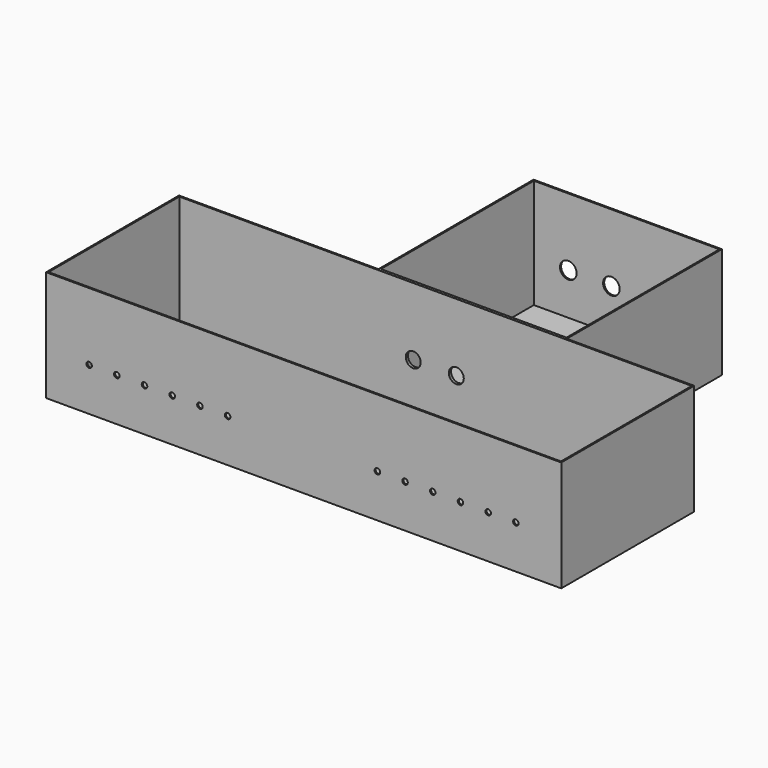
from build123d import *

# Parameters (mm, degrees)
F0_W      = 930
F0_H      = 300
F2_DEPTH  = 200
F3_T      = -2.5
F1_W      = 340
F1_H      = 350
F4_DEPTH  = 200
F5_T      = -2.5
F6_R      = 5
F7_DEPTH  = 25
F8_R      = 13.5
F9_DEPTH  = 25
F10_R     = 15
F11_DEPTH = 25


# Not quite as in the source:
# - a feature names something its author has since deleted; it is built from what else it names


with BuildPart() as f2:
    # F0 (on Top) → F2 (new body)
    with BuildSketch(Plane.XY):
        Rectangle(F0_W, F0_H)
    extrude(amount=F2_DEPTH)

    # F3
    f3_openings = [f2.faces().sort_by_distance(p)[0] for p in [
        (0, 0, 200),
    ]]
    offset(amount=F3_T, openings=f3_openings)

    # F6 (on face) → F7 (cut)
    with BuildSketch(Plane.XZ.offset(150)):
        with Locations((133, 78.065)):
            Circle(F6_R)
        with Locations((183, 78.065)):
            Circle(F6_R)
        with Locations((233, 78.065)):
            Circle(F6_R)
        with Locations((283, 78.065)):
            Circle(F6_R)
        with Locations((383, 78.065)):
            Circle(F6_R)
        with Locations((333, 78.065)):
            Circle(F6_R)
        with Locations((-137.319, 78.065)):
            Circle(F6_R)
        with Locations((-187.319, 78.065)):
            Circle(F6_R)
        with Locations((-237.319, 78.065)):
            Circle(F6_R)
        with Locations((-287.319, 78.065)):
            Circle(F6_R)
        with Locations((-337.319, 78.065)):
            Circle(F6_R)
        with Locations((-387.319, 78.065)):
            Circle(F6_R)
    extrude(amount=-F7_DEPTH, mode=Mode.SUBTRACT)


with BuildPart() as f4:
    # F1 (on Top) → F4 (new body)
    with BuildSketch(Plane.XY):
        with Locations((65, 325)):
            Rectangle(F1_W, F1_H)
    extrude(amount=F4_DEPTH)

    # F5
    f5_openings = [f4.faces().sort_by_distance(p)[0] for p in [
        (65, 325, 200),
    ]]
    offset(amount=F5_T, openings=f5_openings)


with BuildPart() as f9_tool:
    # F8 (on face) → F9 (new body)
    with BuildSketch(Plane.XZ.offset(-147.5)):
        with Locations((37.505, 78.065)):
            Circle(F8_R)
        with Locations((-40.25, 78.065)):
            Circle(F8_R)
    extrude(amount=-F9_DEPTH)


with BuildPart() as f2_1:
    add(f2.part)

    # F9: cut by f9_tool
    add(f9_tool.part, mode=Mode.SUBTRACT)


with BuildPart() as f4_1:
    add(f4.part)

    # F9: cut by f9_tool
    add(f9_tool.part, mode=Mode.SUBTRACT)

    # F10 (on face) → F11 (cut)
    with BuildSketch(Plane(origin=(0, 500, 0), x_dir=(-1, 0, 0), z_dir=(0, 1, 0))):
        with Locations((-37.505, 78.065)):
            Circle(F10_R)
        with Locations((40.25, 78.065)):
            Circle(F10_R)
    extrude(amount=-F11_DEPTH, mode=Mode.SUBTRACT)


solid = Compound([f2_1.part, f4_1.part])
